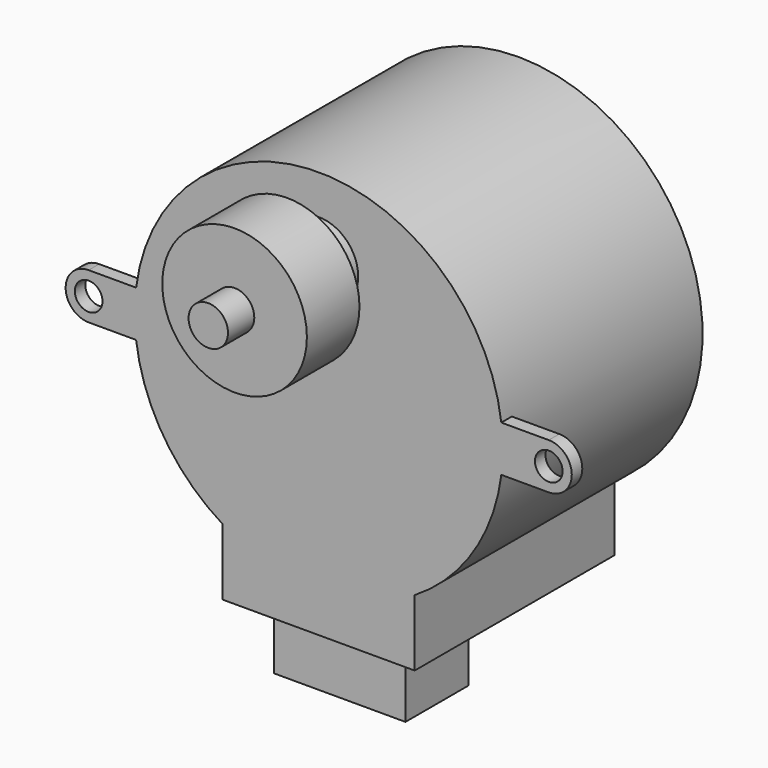
from build123d import *

# Parameters (mm, degrees)
F1_DEPTH  = 19
F2_R      = 3
F3_DEPTH  = 3
F4_R      = 1.5
F5_DEPTH  = 7.5
F6_R      = 1.05
F7_DEPTH  = 1
F8_R      = 5.5
F9_DEPTH  = 5
F10_W     = 10
F10_H     = 6
F11_DEPTH = 5


# Not quite as in the source:
# - a pattern or mirror of a feature is missing from the dataset's text; its kind, count and spacing are read off the source's solid


with BuildPart() as f1:
    # F0 (on Front) → F1 (new body)
    with BuildSketch(Plane.XZ):
        with BuildLine():
            Line((7.3, -17), (7.3, -11.9461290802))
            ThreePointArc((7.3, -11.9461290802), (0, 14), (-7.3, -11.9461290802))
            Line((-7.3, -11.9461290802), (-7.3, -17))
            Line((-7.3, -17), (7.3, -17))
        make_face()
    extrude(amount=F1_DEPTH)

    # F2 (on face) → F3 (join)
    with BuildSketch(Plane.XZ.offset(19)):
        with Locations((0, 8)):
            Circle(F2_R)
    extrude(amount=F3_DEPTH)

    # F4 (on face) → F5 (join)
    with BuildSketch(Plane.XZ.offset(22)):
        with Locations((0, 8)):
            Circle(F4_R)
    extrude(amount=F5_DEPTH)

    # F6 (on face) → F7 (join)
    with BuildSketch(Plane.XZ.offset(19)):
        with BuildLine():
            Line((13.8901943831, -1.75), (17.5, -1.75))
            ThreePointArc((17.5, -1.75), (19.25, 0), (17.5, 1.75))
            Line((17.5, 1.75), (13.8901943831, 1.75))
            Line((13.8901943831, 1.75), (13.8901943831, -1.75))
        make_face()
        with Locations((17.5, 0)):
            Circle(F6_R, mode=Mode.SUBTRACT)
    f7 = extrude(amount=-F7_DEPTH)

    # F7_copies: F7 across plane
    add(f7.mirror(Plane(origin=(0, 0, 0), x_dir=(0, 0, -1), z_dir=(-1, 0, 0))))

    # F8 (on face) → F9 (join)
    with BuildSketch(Plane.XZ.offset(22)):
        with Locations((0, 8)):
            Circle(F8_R)
    extrude(amount=F9_DEPTH)

    # F10 (on face) → F11 (join)
    with BuildSketch(Plane(origin=(0, 0, -17), x_dir=(1, 0, 0), z_dir=(0, 0, -1))):
        with Locations((0, 14)):
            Rectangle(F10_W, F10_H)
    extrude(amount=F11_DEPTH)


solid = f1.part
